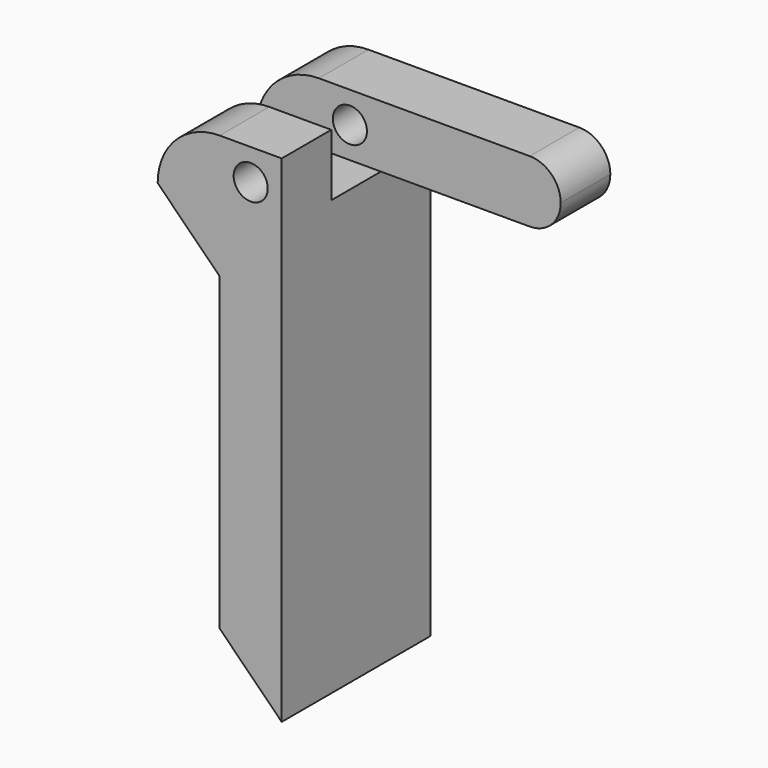
from build123d import *

# Parameters (mm, degrees)
F0_W      = 10
F0_H      = 15
F1_DEPTH  = 5
F2_DEPTH  = 5
F3_R      = 1.375
F4_DEPTH  = 15.001
F5_W      = 5
F5_H      = 5
F6_DEPTH  = 10.001
F7_W      = 5
F7_H      = 5
F8_DEPTH  = 14.5
F9_W      = 5
F9_H      = 15
F10_DEPTH = 30
F11_R     = 2.49999
F12_SIZE  = 4.99999
F13_R     = 5
F14_SIZE  = 4.99999


# Not quite as in the source:
# - a fillet or chamfer is up to 0.001 mm smaller than in the source, because OpenCascade refuses the exact size


with BuildPart() as f1:
    # F0 (on Top) → F1 (new body)
    with BuildSketch(Plane.XY):
        with Locations((-26.6721312702, -21.5040988475)):
            Rectangle(F0_W, F0_H)
    extrude(amount=F1_DEPTH)

    # F2 (add): a face of the model
    f2_faces = [f1.faces().sort_by_distance(p)[0] for p in [
        (-26.6721312702, -21.5040988475, 5),
    ]]
    extrude(f2_faces, amount=F2_DEPTH)

    # F3 (on face) → F4 (cut, through all)
    with BuildSketch(Plane.XZ.offset(29.0040988475)):
        with Locations((-24.1721312702, 7.5)):
            Circle(F3_R)
    extrude(amount=-F4_DEPTH, mode=Mode.SUBTRACT)

    # F5 (on face) → F6 (cut, through all)
    with BuildSketch(Plane.YZ.offset(-21.6721312702)):
        with Locations((-21.5040988475, 7.5)):
            Rectangle(F5_W, F5_H)
    extrude(amount=-F6_DEPTH, mode=Mode.SUBTRACT)

    # F7 (on face) → F8 (join)
    with BuildSketch(Plane.YZ.offset(-21.6721312702)):
        with Locations((-16.5040988475, 7.5)):
            Rectangle(F7_W, F7_H)
    extrude(amount=F8_DEPTH)

    # F9 (on face) → F10 (join)
    with BuildSketch(Plane(origin=(0, 0, 0), x_dir=(1, 0, 0), z_dir=(0, 0, -1))):
        with Locations((-24.1721312702, 21.5040988475)):
            Rectangle(F9_W, F9_H)
    extrude(amount=F10_DEPTH)

    # F11 (radius 2.5 in the source; OpenCascade refuses exactly that, so slightly less here)
    f11_edges = [f1.edges().sort_by_distance(p)[0] for p in [
        (-7.172131, -16.504099, 10),
        (-7.172131, -16.504099, 5),
    ]]
    fillet(f11_edges, radius=F11_R)

    # F12 (size 5 in the source; OpenCascade refuses exactly that, so slightly less here)
    f12_edges = [f1.edges().sort_by_distance(p)[0] for p in [
        (-31.672131, -21.504099, 0),
    ]]
    chamfer(f12_edges, length=F12_SIZE)

    # F13
    f13_edges = [f1.edges().sort_by_distance(p)[0] for p in [
        (-31.672131, -16.504099, 10),
        (-31.672131, -26.504099, 10),
    ]]
    fillet(f13_edges, radius=F13_R)

    # F14 (size 5 in the source; OpenCascade refuses exactly that, so slightly less here)
    f14_edges = [f1.edges().sort_by_distance(p)[0] for p in [
        (-26.672131, -21.504099, -30),
    ]]
    chamfer(f14_edges, length=F14_SIZE)


solid = f1.part
